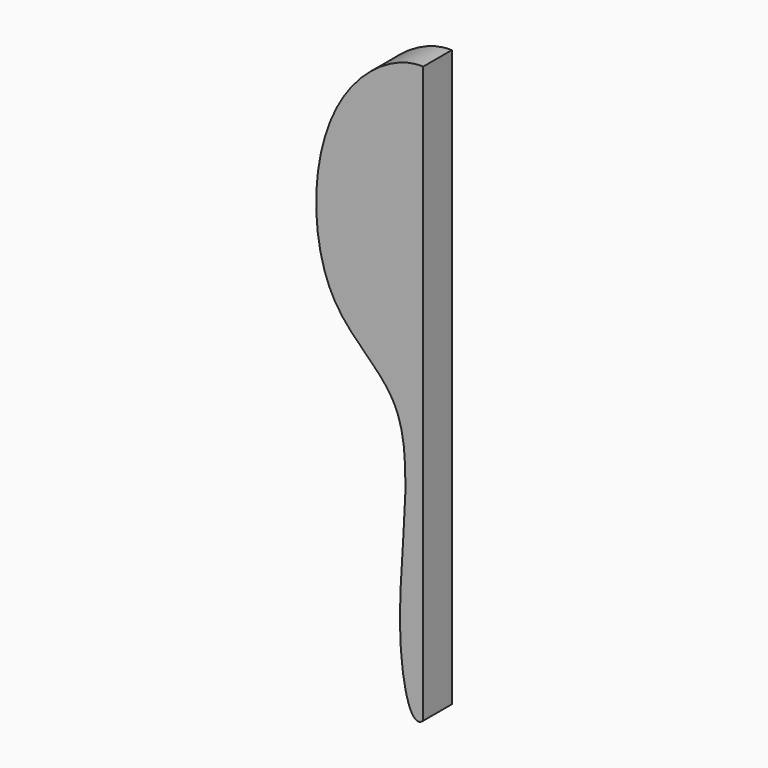
from build123d import *

# Parameters (mm, degrees)
F1_DEPTH = 5.08


with BuildPart() as f1:
    # F0 (on Front) → F1 (new body)
    with BuildSketch(Plane.XZ):
        with BuildLine():
            add(Edge.make_bspline(
                [(0, 0), (-1.8327142489, -1.7439200741), (-5.1525730731, 12.8186221726), (0.6958792682, 39.6423714251), (-16.6003424615, 46.7933249724), (-16.1337743554, 74.1643177975), (-3.6716484874, 82.234367016), (0, 82.098153585)],
                knots=[0, 0, 0, 0, 0.1060356433, 0.2791607625, 0.4052751949, 0.5750112371, 0.6589733151, 0.6589733151, 0.6589733151, 0.6589733151], degree=3))
            Line((0, 0), (0, 82.098153585))
        make_face()
    extrude(amount=F1_DEPTH)


solid = f1.part
